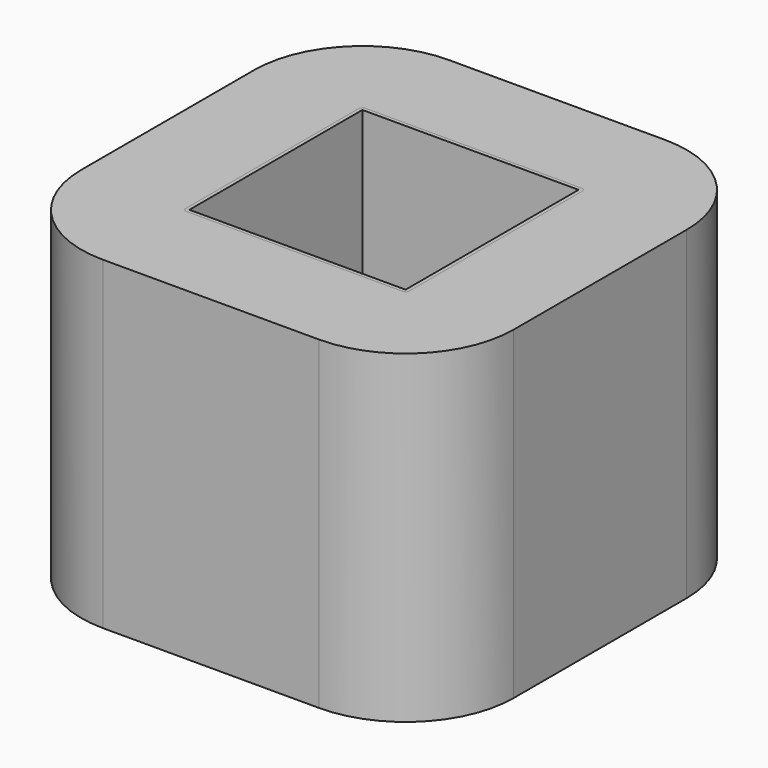
from build123d import *

# Parameters (mm, degrees)
F4_W      = 45.974
F4_H      = 45.974
F5_DEPTH  = 66.675
F6_W      = 44.45
F6_H      = 44.45
F7_DEPTH  = 66.675
F8_R      = 0.762
F9_W      = 88.9
F9_H      = 88.9
F10_DEPTH = 66.675
F11_R     = 22.225
F12_R     = 0.762


# Not quite as in the source:
# - a variable given as a bare number and used for a length is read in inches; the dataset says mm whatever the document's units were


with BuildPart() as f5:
    # F4 (on Top) → F5 (new body)
    with BuildSketch(Plane.XY):
        Rectangle(F4_W, F4_H)
    extrude(amount=F5_DEPTH)

    # F6 (on face) → F7 (cut)
    with BuildSketch(Plane.XY.offset(66.675)):
        Rectangle(F6_W, F6_H)
    extrude(amount=-F7_DEPTH, mode=Mode.SUBTRACT)

    # F8
    f8_edges = [f5.edges().sort_by_distance(p)[0] for p in [
        (-22.987, 22.987, 33.3375),
        (22.987, 22.987, 33.3375),
        (-22.987, -22.987, 33.3375),
        (22.987, -22.987, 33.3375),
    ]]
    fillet(f8_edges, radius=F8_R)


with BuildPart() as f10:
    # F9 (on face) → F10 (new body)
    with BuildSketch(Plane.XY.offset(66.675)):
        Rectangle(F9_W, F9_H)
        Polygon((-22.987, 22.225), (-22.987, 22.987), (-22.225, 22.987), (22.225, 22.987), (22.987, 22.987), (22.987, 22.225), (22.987, -22.225), (22.987, -22.987), (22.225, -22.987), (-22.225, -22.987), (-22.987, -22.987), (-22.987, -22.225), align=None, mode=Mode.SUBTRACT)
    extrude(amount=-F10_DEPTH)

    # F11
    f11_edges = [f10.edges().sort_by_distance(p)[0] for p in [
        (-44.45, 44.45, 33.3375),
        (-44.45, -44.45, 33.3375),
        (44.45, -44.45, 33.3375),
        (44.45, 44.45, 33.3375),
    ]]
    fillet(f11_edges, radius=F11_R)

    # F12
    f12_edges = [f10.edges().sort_by_distance(p)[0] for p in [
        (-22.987, 22.987, 33.3375),
        (22.987, 22.987, 33.3375),
        (22.987, -22.987, 33.3375),
        (-22.987, -22.987, 33.3375),
    ]]
    fillet(f12_edges, radius=F12_R)


solid = Compound([f5.part, f10.part])
